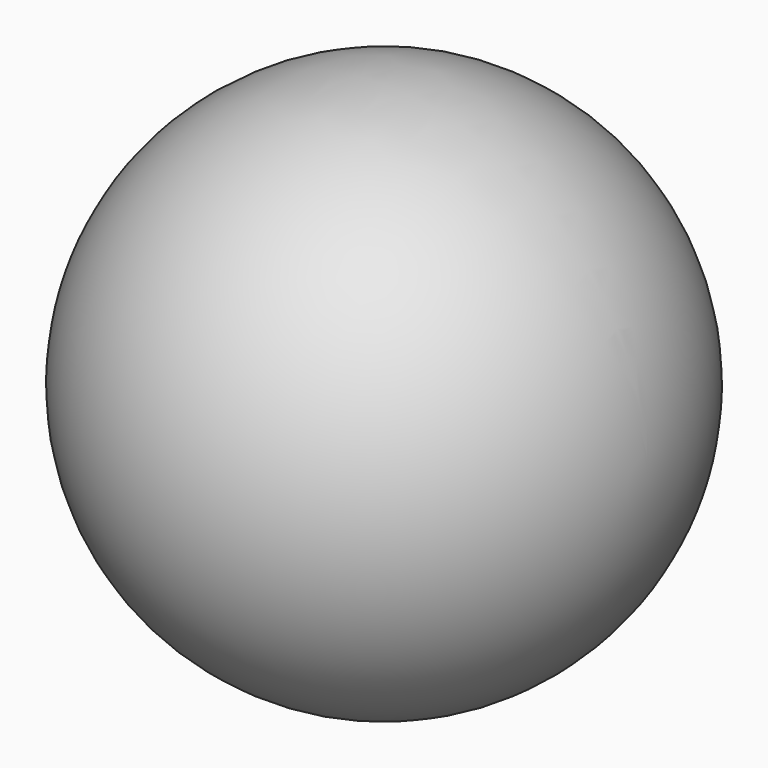
from build123d import *


with BuildPart() as f1:
    # F0 (on Front) → F1 (revolve)
    with BuildSketch(Plane.XZ):
        with BuildLine():
            Line((0, 0), (29.1299579932, 0))
            ThreePointArc((29.1299579932, 0), (0, 29.1299579932), (-29.1299579932, 0))
            Line((-29.1299579932, 0), (0, 0))
        make_face()
    revolve(axis=Axis((4.6588722616, 0, 0), (-1, 0, 0)))


solid = f1.part
